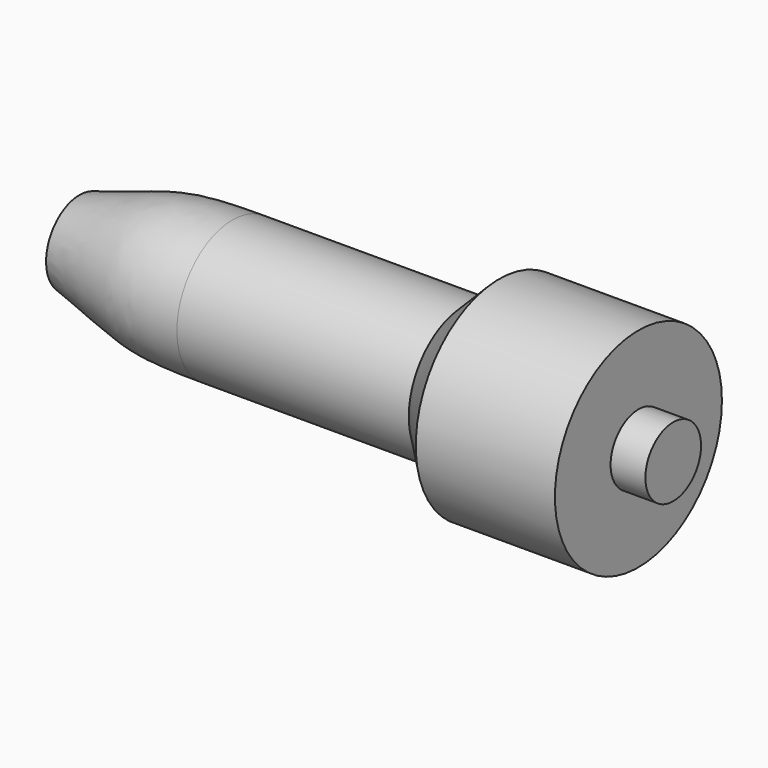
from build123d import *

# Parameters (mm, degrees)
F0_W     = 100
F0_H     = 30
F3_R     = 45
F3_R_2   = 30
F4_DEPTH = 75
F5_SIZE  = 14.99999
F7_R     = 15
F8_DEPTH = 15


# Not quite as in the source:
# - a fillet or chamfer is up to 0.001 mm smaller than in the source, because OpenCascade refuses the exact size


with BuildPart() as f1:
    # F0 (on Front) → F1 (revolve)
    with BuildSketch(Plane.XZ):
        with BuildLine():
            Line((0, 18), (0, 0))
            Line((0, 0), (50, 0))
            Line((50, 0), (50, 30))
            add(Edge.make_bspline(
                [(-16, 18), (17.3213258386, 27.5211501867), (16.1499090196, 30), (50, 30)],
                knots=[0, 0, 0, 0, 67.082039325, 67.082039325, 67.082039325, 67.082039325], degree=3))
            Line((-16, 18), (0, 18))
        make_face()
        with Locations((100, 15)):
            Rectangle(F0_W, F0_H)
    revolve(axis=Axis((25, 0, 0), (-1, 0, 0)))

    # F3 (on offset) → F4 (join)
    with BuildSketch(Plane.YZ.offset(150)):
        Circle(F3_R)
        Circle(F3_R_2, mode=Mode.SUBTRACT)
        Circle(F3_R_2)
    extrude(amount=F4_DEPTH)

    # F5 (size 15 in the source; OpenCascade refuses exactly that, so slightly less here)
    f5_edges = [f1.edges().sort_by_distance(p)[0] for p in [
        (150, -45, 0),
    ]]
    chamfer(f5_edges, length=F5_SIZE)

    # F7 (on offset) → F8 (join)
    with BuildSketch(Plane.YZ.offset(225)):
        Circle(F7_R)
    extrude(amount=F8_DEPTH)


solid = f1.part
